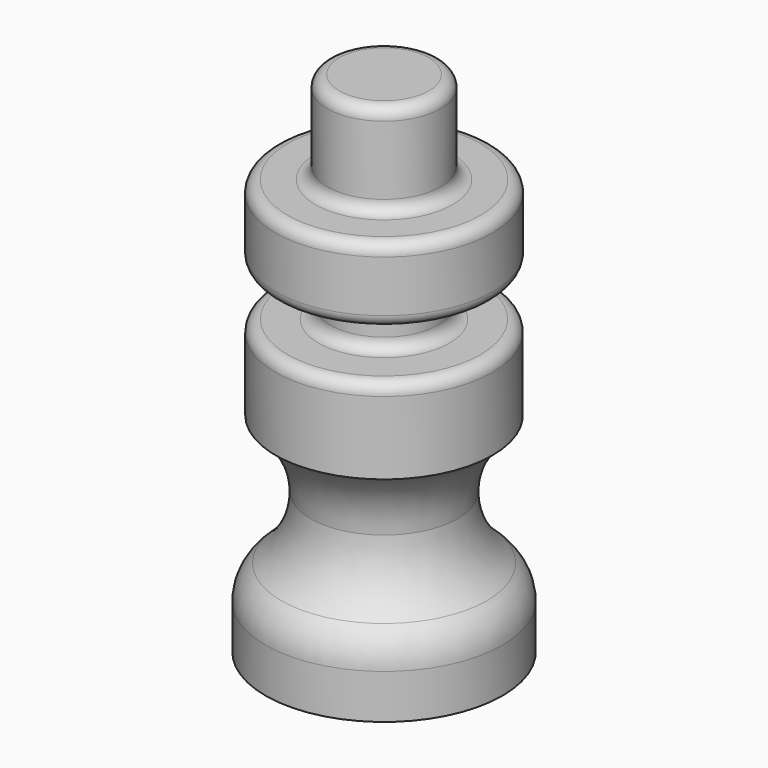
from build123d import *

# Parameters (mm, degrees)
F0_R      = 50.7207222374
F1_DEPTH  = 38.1
F2_R      = 31.5363101215
F3_DEPTH  = 90.17
F5_START  = 89.154
F4_R      = 46.3942774272
F5_DEPTH  = 36.322
F7_START  = 121.158
F6_R      = 22.9400039182
F7_DEPTH  = 29.718
F9_START  = 145.796
F8_R      = 46.4761093374
F9_DEPTH  = 32.258
F11_START = 176.53
F10_R     = 24.2550849765
F11_DEPTH = 41.148
F12_R     = 19.05
F14_R     = 5.08
F15_R     = 5.08
F16_R     = 5.08


# Not quite as in the source:
# - a fillet or chamfer that OpenCascade refuses, or shapes differently, is made with other operations: its cross-section is extruded or revolved along the edge and cut away or added


with BuildPart() as f1:
    # F0 (on Top) → F1 (new body)
    with BuildSketch(Plane.XY):
        Circle(F0_R)
    extrude(amount=F1_DEPTH)

    # F2 (on Top) → F3 (join)
    with BuildSketch(Plane.XY):
        Circle(F2_R)
    extrude(amount=F3_DEPTH)

    # F4 (on Top) → F5 (join)
    with BuildSketch(Plane.XY.offset(F5_START)):
        Circle(F4_R)
    extrude(amount=F5_DEPTH)

    # F6 (on Top) → F7 (join)
    with BuildSketch(Plane.XY.offset(F7_START)):
        Circle(F6_R)
    extrude(amount=F7_DEPTH)

    # F8 (on Top) → F9 (join)
    with BuildSketch(Plane.XY.offset(F9_START)):
        Circle(F8_R)
    extrude(amount=F9_DEPTH)

    # F10 (on Top) → F11 (join)
    with BuildSketch(Plane.XY.offset(F11_START)):
        Circle(F10_R)
    extrude(amount=F11_DEPTH)

    # F12
    f12_edges = [f1.edges().sort_by_distance(p)[0] for p in [
        (-50.720722, 0, 38.1),
    ]]
    fillet(f12_edges, radius=F12_R)

    # F13: fillet of radius 35.179 on 3 edges, made by hand

    # F13_s1 → F13_t2 (revolve)
    with BuildSketch(Plane.XZ):
        with BuildLine():
            ThreePointArc((31.5363101215, 60.437843028), (35.470825407, 76.6039871547), (46.3942774272, 89.154))
            Line((46.3942774272, 89.154), (31.5363101215, 89.154))
            Line((31.5363101215, 89.154), (31.5363101215, 60.437843028))
        make_face()
    revolve(axis=Axis((0, 0, 89.154), (0, 0, -1)))

    # F13_s3 → F13_t4 (revolve)
    with BuildSketch(Plane.XZ):
        with BuildLine():
            ThreePointArc((43.9814673957, 33.5878146104), (34.7988888446, 45.6389043931), (31.5363101215, 60.4343122576))
            Line((31.5363101215, 60.4343122576), (28.0184101215, 60.4343122576))
            Line((28.0184101215, 60.4343122576), (28.0184101215, 38.1))
            Line((28.0184101215, 38.1), (31.5363101215, 34.5821))
            ThreePointArc((31.5363101215, 34.5821), (31.6707222374, 34.5821), (41.7080831232, 30.9031648457))
            Line((41.7080831232, 30.9031648457), (43.9814673957, 33.5878146104))
        make_face()
    revolve(axis=Axis((0, 0, 38.1), (0, 0, -1)))

    # F14
    f14_edges = [f1.edges().sort_by_distance(p)[0] for p in [
        (-46.394277, 0, 125.476),
    ]]
    fillet(f14_edges, radius=F14_R)

    # F15
    f15_edges = [f1.edges().sort_by_distance(p)[0] for p in [
        (22.940004, 0, 135.636),
        (-22.940004, 0, 145.796),
        (-22.940004, 0, 125.476),
    ]]
    fillet(f15_edges, radius=F15_R)

    # F16
    f16_edges = [f1.edges().sort_by_distance(p)[0] for p in [
        (-46.476109, 0, 145.796),
        (-46.476109, 0, 178.054),
        (-24.255085, 0, 178.054),
        (24.255085, 0, 197.866),
        (-24.255085, 0, 217.678),
    ]]
    fillet(f16_edges, radius=F16_R)


solid = f1.part
